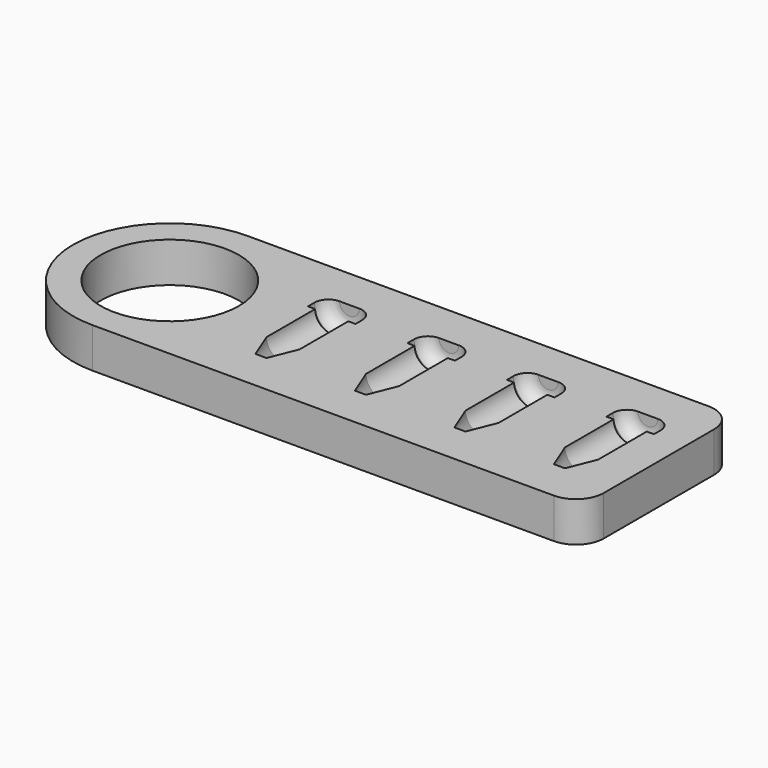
from build123d import *

# Parameters (mm, degrees)
F0_R         = 12.5
F1_DEPTH     = 7.25
F7_TEXT_SIZE = 5.5555555556
F8_DEPTH     = 1


# Not quite as in the source:
# - Text() gives the source's letters only with a copy of the font that has no kerning and outlines rounded to 1/6400 em; it was checked with that copy


with BuildPart() as f1:
    # F0 (on Top) → F1 (new body)
    with BuildSketch(Plane.XY):
        with BuildLine():
            ThreePointArc((0, 17.5), (5.1256313292, 5.1256313292), (17.5, 0))
            Line((17.5, 0), (101, 0))
            ThreePointArc((101, 0), (104.5355339059, 1.4644660941), (106, 5))
            Line((106, 5), (106, 30))
            ThreePointArc((106, 30), (104.5355339059, 33.5355339059), (101, 35))
            Line((101, 35), (17.5, 35))
            ThreePointArc((17.5, 35), (5.1256313292, 29.8743686708), (0, 17.5))
        make_face()
        with Locations((17.5, 17.5)):
            Circle(F0_R, mode=Mode.SUBTRACT)
    extrude(amount=F1_DEPTH)

    # F2 (on face) → F3 (revolve, cut)
    with BuildSketch(Plane.XY.offset(7.25)):
        with BuildLine():
            Line((42, 10.5), (42, 7.5))
            Line((42, 7.5), (43, 7.5))
            Line((43, 7.5), (45, 12.5))
            Line((45, 12.5), (45, 23.5))
            Line((45, 23.5), (46.3, 23.5))
            Line((46.3, 23.5), (46.3, 25))
            ThreePointArc((46.3, 25), (45.567766953, 26.767766953), (43.8, 27.5))
            Line((43.8, 27.5), (42, 27.5))
            Line((42, 27.5), (42, 23.5))
            Line((42, 23.5), (42, 10.5))
        make_face()
    revolve(axis=Axis((42, 15.5, 7.25), (0, 1, 0)), mode=Mode.SUBTRACT)

    # F2 (on face) → F4 (revolve, cut)
    with BuildSketch(Plane.XY.offset(7.25)):
        with BuildLine():
            Line((60, 10.5), (60, 7.5))
            Line((60, 7.5), (61, 7.5))
            Line((61, 7.5), (63, 12.5))
            Line((63, 12.5), (63, 23.5))
            Line((63, 23.5), (64.3, 23.5))
            Line((64.3, 23.5), (64.3, 25))
            ThreePointArc((64.3, 25), (63.567766953, 26.767766953), (61.8, 27.5))
            Line((61.8, 27.5), (60, 27.5))
            Line((60, 27.5), (60, 23.5))
            Line((60, 23.5), (60, 10.5))
        make_face()
    revolve(axis=Axis((60, 15.5, 7.25), (0, 1, 0)), mode=Mode.SUBTRACT)

    # F2 (on face) → F5 (revolve, cut)
    with BuildSketch(Plane.XY.offset(7.25)):
        with BuildLine():
            Line((78, 12.5), (78, 7.5))
            Line((78, 7.5), (79, 7.5))
            Line((79, 7.5), (81, 12.5))
            Line((81, 12.5), (81, 23.5))
            Line((81, 23.5), (82.3, 23.5))
            Line((82.3, 23.5), (82.3, 25))
            ThreePointArc((82.3, 25), (81.567766953, 26.767766953), (79.8, 27.5))
            Line((79.8, 27.5), (78, 27.5))
            Line((78, 27.5), (78, 23.5))
            Line((78, 23.5), (78, 12.5))
        make_face()
    revolve(axis=Axis((78, 18, 7.25), (0, -1, 0)), mode=Mode.SUBTRACT)

    # F2 (on face) → F6 (revolve, cut)
    with BuildSketch(Plane.XY.offset(7.25)):
        with BuildLine():
            Line((96, 10.5), (96, 7.5))
            Line((96, 7.5), (97, 7.5))
            Line((97, 7.5), (99, 12.5))
            Line((99, 12.5), (99, 23.5))
            Line((99, 23.5), (100.3, 23.5))
            Line((100.3, 23.5), (100.3, 25))
            ThreePointArc((100.3, 25), (99.567766953, 26.767766953), (97.8, 27.5))
            Line((97.8, 27.5), (96, 27.5))
            Line((96, 27.5), (96, 23.5))
            Line((96, 23.5), (96, 10.5))
        make_face()
    revolve(axis=Axis((96, 15.5, 7.25), (0, 1, 0)), mode=Mode.SUBTRACT)

    # F7 (on face) → F8 (cut)
    with BuildSketch(Plane(origin=(0, 0, 0), x_dir=(1, 0, 0), z_dir=(0, 0, -1))):
        with Locations((30, -9)):
            Text('797', F7_TEXT_SIZE, font='Open Sans', text_align=(TextAlign.LEFT, TextAlign.BOTTOM))
    extrude(amount=-F8_DEPTH, mode=Mode.SUBTRACT)


solid = f1.part
